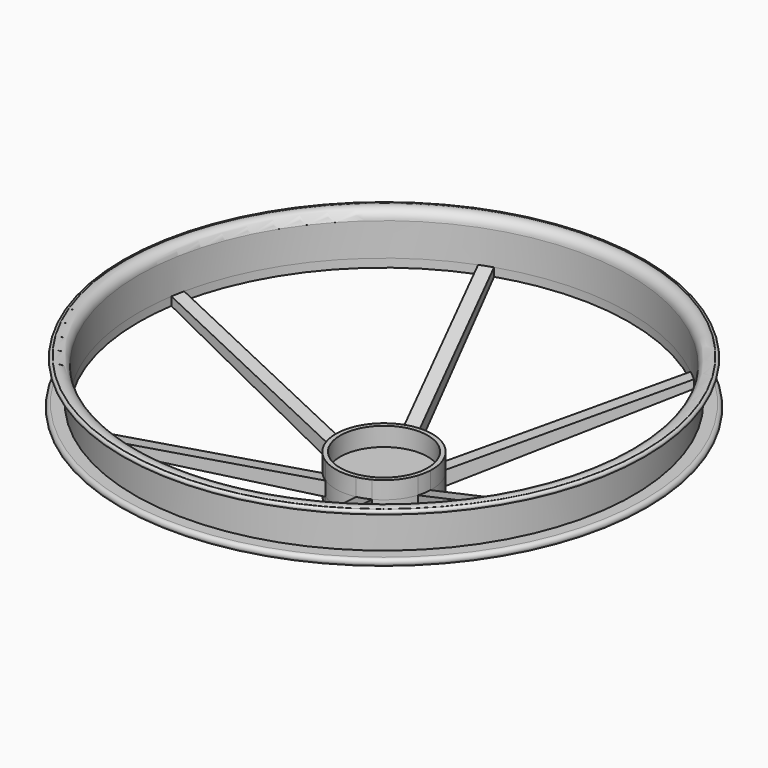
from build123d import *
from build123d import SkipClean  # not in build123d's __all__

# Parameters (mm, degrees)
F5_DEPTH = 25


with BuildPart() as f3:
    # F2 (on offset) → F3 (revolve)
    with BuildSketch(Plane.XZ.offset(65)):
        with BuildLine():
            Line((-65, -15.9252075107), (-65, -14))
            Line((-65, -14), (-75, -14))
            Line((-75, -14), (-75, -9.7358990461))
            Line((-75, -9.7358990461), (-76, -9.7358990461))
            Line((-76, -9.7358990461), (-76, -13.6956521739))
            Line((-76, -13.6956521739), (-121, 0))
            Line((-121, 0), (-121, 7.5354827568))
            ThreePointArc((-121, 7.5354827568), (-122.0045964257, 9.3632036252), (-124.0860596299, 9.4946892932))
            ThreePointArc((-124.0860596299, 9.4946892932), (-124.7034612564, 9.1920763963), (-124.4362071157, 8.558566682))
            Line((-124.4362071157, 8.558566682), (-121.8917220831, 7.4391760863))
            Line((-121.8917220831, 7.4391760863), (-121.8917220831, 0))
            Line((-121.8917220831, 0), (-124.4616806507, 0))
            ThreePointArc((-124.4616806507, 0), (-125.2788653783, -0.8218546839), (-124.452367425, -1.6343429199))
            Line((-124.452367425, -1.6343429199), (-121.8917220831, -1.6343429199))
            Line((-121.8917220831, -1.6343429199), (-76, -16.9519204646))
            Line((-76, -16.9519204646), (-76, -18.5886826366))
            Line((-76, -18.5886826366), (-75, -18.5886826366))
            Line((-75, -18.5886826366), (-75.03588984, -15.9252075107))
            Line((-75.03588984, -15.9252075107), (-65, -15.9252075107))
        make_face()
    revolve(axis=Axis((-65, -65, -7), (0, 0, -1)))

    # F4 (on Top) → F5 (cut)
    with BuildSketch(Plane.XY):
        with BuildLine():
            ThreePointArc((-56.80714849, -57.6598920897), (-54.643510446, -61.2928280161), (-54.0101980565, -65.4735538439))
            Line((-54.0101980565, -65.4735538439), (-9.6349567528, -73.5417788684))
            ThreePointArc((-9.6349567528, -73.5417788684), (-12.2571425277, -46.1203552561), (-27.6322400034, -23.2639183339))
            Line((-27.6322400034, -23.2639183339), (-56.80714849, -57.6598920897))
        make_face()
        with BuildLine():
            Line((-70.0847913129, -55.2457754124), (-85.2851241301, -12.7815766321))
            ThreePointArc((-85.2851241301, -12.7815766321), (-107.7216806988, -28.7631679328), (-119.8283869755, -53.5066113935))
            Line((-119.8283869755, -53.5066113935), (-75.4531456718, -61.574836418))
            ThreePointArc((-75.4531456718, -61.574836418), (-73.3887498913, -57.8846029442), (-70.0847913129, -55.2457754124))
        make_face()
        with BuildLine():
            ThreePointArc((-29.9200808829, -21.3233555005), (-54.9788232265, -9.8835231888), (-82.460626979, -11.7705297274))
            Line((-82.460626979, -11.7705297274), (-67.2602941618, -54.2347285077))
            ThreePointArc((-67.2602941618, -54.2347285077), (-63.0322603373, -54.1774309603), (-59.0949893694, -55.7193292563))
            Line((-59.0949893694, -55.7193292563), (-29.9200808829, -21.3233555005))
        make_face()
        with BuildLine():
            ThreePointArc((-44.7148758699, -117.2184233679), (-22.2783193012, -101.2368320672), (-10.1716130245, -76.4933886065))
            Line((-10.1716130245, -76.4933886065), (-54.5468543282, -68.425163582))
            ThreePointArc((-54.5468543282, -68.425163582), (-56.6112501087, -72.1153970558), (-59.9152086871, -74.7542245876))
            Line((-59.9152086871, -74.7542245876), (-44.7148758699, -117.2184233679))
        make_face()
        with BuildLine():
            Line((-70.9050106306, -74.2806707437), (-100.0799191171, -108.6766444995))
            ThreePointArc((-100.0799191171, -108.6766444995), (-75.0211767735, -120.1164768112), (-47.539373021, -118.2294702726))
            Line((-47.539373021, -118.2294702726), (-62.7397058382, -75.7652714923))
            ThreePointArc((-62.7397058382, -75.7652714923), (-66.9677396627, -75.8225690397), (-70.9050106306, -74.2806707437))
        make_face()
        with BuildLine():
            ThreePointArc((-120.3650432472, -56.4582211316), (-117.7428574723, -83.8796447439), (-102.3677599966, -106.7360816661))
            Line((-102.3677599966, -106.7360816661), (-73.19285151, -72.3401079103))
            ThreePointArc((-73.19285151, -72.3401079103), (-75.356489554, -68.7071719839), (-75.9898019435, -64.5264461561))
            Line((-75.9898019435, -64.5264461561), (-120.3650432472, -56.4582211316))
        make_face()
    with SkipClean():  # cleaning this boolean's faces spoils the solid; the shape is the same uncleaned
        extrude(amount=-F5_DEPTH, mode=Mode.SUBTRACT)


solid = f3.part
